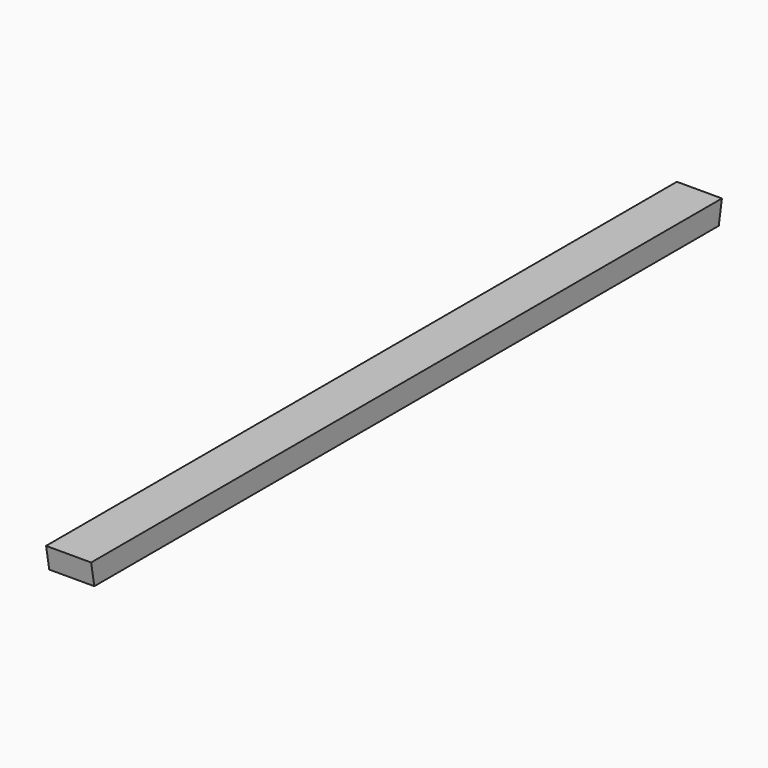
from build123d import *

# Parameters (mm, degrees)
F0_W     = 40
F0_H     = 20
F1_DEPTH = 700
F2_SIZE2 = 3.52653
F2_SIZE  = 19.99999
F3_SIZE2 = 3.52653
F3_SIZE  = 19.99999


# Not quite as in the source:
# - a fillet or chamfer is up to 0.001 mm smaller than in the source, because OpenCascade refuses the exact size


with BuildPart() as f1:
    # F0 (on Front) → F1 (new body)
    with BuildSketch(Plane.XZ):
        with Locations((20, 10)):
            Rectangle(F0_W, F0_H)
    extrude(amount=F1_DEPTH)

    # F2 (size 20 and 3.5265396142 in the source; OpenCascade refuses exactly that, so slightly less here)
    f2_edges = [f1.edges().sort_by_distance(p)[0] for p in [
        (20, -700, 0),
    ]]
    f2_side = f1.faces().sort_by_distance((20, -700, 10))[0]
    chamfer(f2_edges, length=F2_SIZE, length2=F2_SIZE2, reference=f2_side)

    # F3 (size 20 and 3.5265396142 in the source; OpenCascade refuses exactly that, so slightly less here)
    f3_edges = [f1.edges().sort_by_distance(p)[0] for p in [
        (20, 0, 0),
    ]]
    f3_side = f1.faces().sort_by_distance((20, 0, 10))[0]
    chamfer(f3_edges, length=F3_SIZE, length2=F3_SIZE2, reference=f3_side)


solid = f1.part
